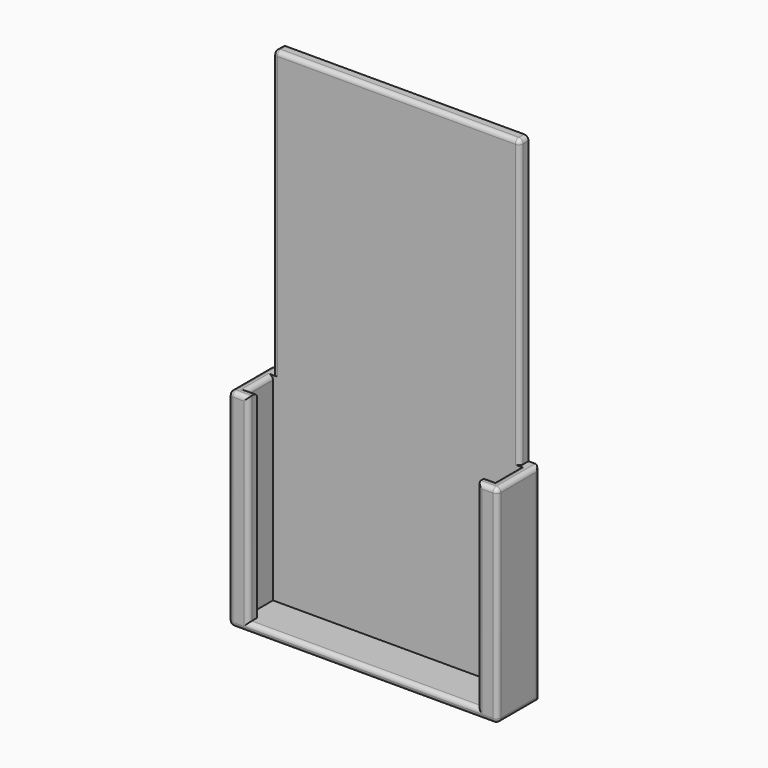
from build123d import *

# Parameters (mm, degrees)
F0_W     = 61
F0_H     = 12
F0_W_2   = 56
F0_H_2   = 7
F1_DEPTH = 45
F2_W     = 52
F2_H     = 45
F3_DEPTH = 3
F4_W     = 61
F4_H     = 12
F5_DEPTH = 2
F6_W     = 56
F6_H     = 2.5
F7_DEPTH = 65
F8_R     = 0.99999
F9_R     = 0.99999


# Not quite as in the source:
# - a fillet or chamfer is up to 0.001 mm smaller than in the source, because OpenCascade refuses the exact size


with BuildPart() as f1:
    # F0 (on Top) → F1 (new body)
    with BuildSketch(Plane.XY):
        Rectangle(F0_W, F0_H)
        Rectangle(F0_W_2, F0_H_2, mode=Mode.SUBTRACT)
    extrude(amount=F1_DEPTH)

    # F2 (on face) → F3 (cut)
    with BuildSketch(Plane.XZ.offset(6)):
        with Locations((0, 22.5)):
            Rectangle(F2_W, F2_H)
    extrude(amount=-F3_DEPTH, mode=Mode.SUBTRACT)

    # F4 (on face) → F5 (join)
    with BuildSketch(Plane(origin=(0, 0, 0), x_dir=(1, 0, 0), z_dir=(0, 0, -1))):
        Rectangle(F4_W, F4_H)
    extrude(amount=F5_DEPTH)

    # F6 (on face) → F7 (join)
    with BuildSketch(Plane.XY.offset(45)):
        with Locations((0, 4.75)):
            Rectangle(F6_W, F6_H)
    extrude(amount=F7_DEPTH)

    # F8 (radius 1 in the source; OpenCascade refuses exactly that, so slightly less here)
    f8_edges = [f1.edges().sort_by_distance(p)[0] for p in [
        (-26, -6, 22.5),
        (0, -6, 0),
        (26, -6, 22.5),
        (28.25, -6, 45),
        (30.5, -6, 21.5),
        (0, -6, -2),
        (-30.5, -6, 21.5),
        (-28.25, -6, 45),
        (-28, 0, 45),
        (28, 0, 45),
        (27, -3.5, 45),
        (-27, -3.5, 45),
        (-30.5, 0, 45),
        (30.5, 0, 45),
        (30.5, 6, 21.5),
        (30.5, 0, -2),
        (-30.5, 6, 21.5),
        (-30.5, 0, -2),
        (0, 3.5, 110),
    ]]
    fillet(f8_edges, radius=F8_R)

    # F9 (radius 1 in the source; OpenCascade refuses exactly that, so slightly less here)
    f9_edges = [f1.edges().sort_by_distance(p)[0] for p in [
        (-28, 3.5, 77.000005),
        (28, 3.5, 77.000005),
    ]]
    fillet(f9_edges, radius=F9_R)


solid = f1.part
